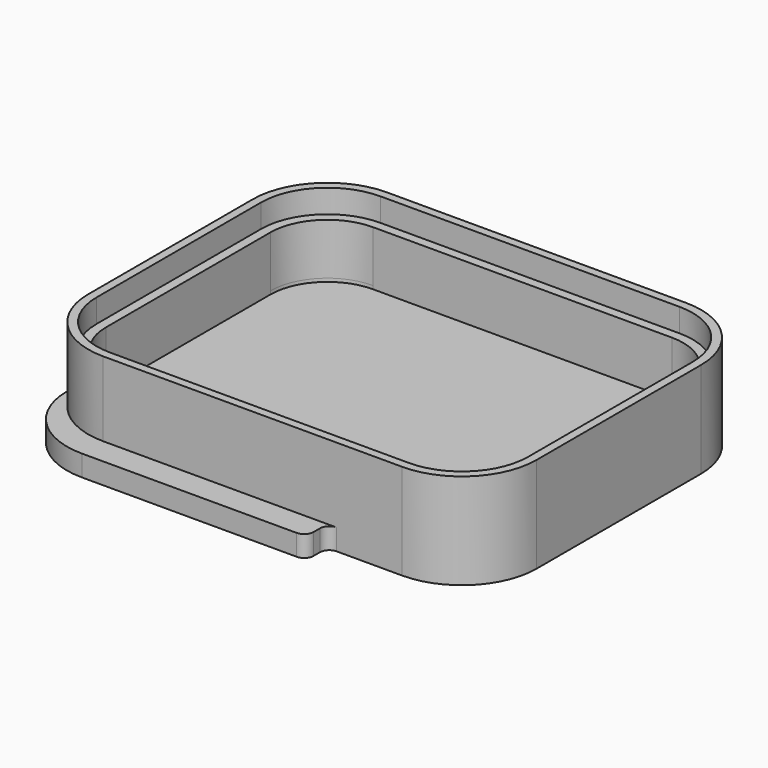
from build123d import *

# Parameters (mm, degrees)
F1_DEPTH     = 10.25
F3_DEPTH     = 2.25
F4_R         = 1
F5_T         = 1.9
F5_T3_DEPTH  = 4.8
F5_T5_DEPTH  = 27.8
F5_T8_ANGLE  = 90.000000001
F5_T10_ANGLE = 90.000000001
F7_DEPTH     = 2.5


# Not quite as in the source:
# - a shell that OpenCascade refuses in one call is made with other operations: the cavity is built on its own and cut out


with BuildPart() as f1:
    # F0 (on Top) → F1 (new body)
    with BuildSketch(Plane.XY):
        with BuildLine():
            Line((16, 19), (-16, 19))
            ThreePointArc((-16, 19), (-21.6568542495, 16.6568542495), (-24, 11))
            Line((-24, 11), (-24, -11))
            ThreePointArc((-24, -11), (-21.6568542495, -16.6568542495), (-16, -19))
            Line((-16, -19), (16, -19))
            ThreePointArc((16, -19), (21.6568542495, -16.6568542495), (24, -11))
            Line((24, -11), (24, 11))
            ThreePointArc((24, 11), (21.6568542495, 16.6568542495), (16, 19))
        make_face()
    extrude(amount=F1_DEPTH)

    # F2 (on Top) → F3 (join)
    with BuildSketch(Plane.XY):
        with BuildLine():
            Line((8, 21.85), (-16, 21.85))
            ThreePointArc((-16, 21.85), (-21.6568542495, 19.5068542495), (-24, 13.85))
            Line((-24, 13.85), (-24, -13.85))
            ThreePointArc((-24, -13.85), (-21.6568542495, -19.5068542495), (-16, -21.85))
            Line((-16, -21.85), (8, -21.85))
            Line((8, -21.85), (8, 21.85))
        make_face()
    extrude(amount=F3_DEPTH)

    # F4
    f4_edges = [f1.edges().sort_by_distance(p)[0] for p in [
        (8, 21.85, 1.125),
        (8, 19, 1.125),
        (8, -19, 1.125),
        (8, -21.85, 1.125),
    ]]
    fillet(f4_edges, radius=F4_R)

    # F5: shell of thickness 1.9, made by hand


with BuildPart() as f5_core1:
    # F5_t2: copy of F1
    add(f1.part)

    # the walls: a layer under each face that stays
    f5_faces = [f5_core1.faces().sort_by_distance(p)[0] for p in [
        (0, 19, 5.125),
        (0, 0, 0),
        (8.2928932188, 19.2928932188, 1.125),
        (21.6568542495, 16.6568542495, 5.125),
        (-18.5, 20.0416666667, 2.25),
        (-21.6568542495, 16.6568542495, 6.25),
        (8, 20.425, 1.125),
        (24, 0, 5.125),
        (21.6568542495, -16.6568542495, 5.125),
        (-4.5, 21.85, 1.125),
        (0, -19, 5.125),
        (-21.6568542495, 19.5068542495, 1.125),
        (8.2928932188, -19.2928932188, 1.125),
        (-24, 0, 5.125),
        (8, -20.425, 1.125),
        (-21.6568542495, -19.5068542495, 1.125),
        (-4.5, -21.85, 1.125),
        (-21.6568542495, -16.6568542495, 6.25),
        (-18.5, -20.0416666667, 2.25),
    ]]
    thicken(f5_faces, amount=-F5_T, mode=Mode.SUBTRACT)

    # F5_s4 → F5_t3 (cut)
    with BuildSketch(Plane.YZ.offset(6.1)):
        Polygon((19.019, 2.269), (17.1, 2.25), (17.1, 0.35), (19, 0.35), align=None)
        Polygon((-19.019, 2.269), (-17.1, 2.25), (-17.1, 0.35), (-19, 0.35), align=None)
    extrude(amount=F5_T3_DEPTH, mode=Mode.SUBTRACT)

    # F5_s6 → F5_t5 (cut)
    with BuildSketch(Plane.YZ.offset(-17.9)):
        Polygon((19.019, 2.269), (17.1, 2.25), (17.1, 0.35), (19, 0.35), align=None)
        Polygon((-19.019, 2.269), (-17.1, 2.25), (-17.1, 0.35), (-19, 0.35), align=None)
    extrude(amount=F5_T5_DEPTH, mode=Mode.SUBTRACT)

    # F5_s7 → F5_t8 (revolve, cut)
    with BuildSketch(Plane.XZ.offset(-11)):
        Polygon((-24.019, 2.269), (-24, 0.35), (-22.1, 0.35), (-22.1, 2.25), align=None)
    revolve(axis=Axis((-16, 11, 2.25), (0, 0, -1)), revolution_arc=F5_T8_ANGLE, mode=Mode.SUBTRACT)

    # F5_s9 → F5_t10 (revolve, cut)
    with BuildSketch(Plane.YZ.offset(-16)):
        Polygon((-19.019, 2.269), (-17.1, 2.25), (-17.1, 0.35), (-19, 0.35), align=None)
    revolve(axis=Axis((-16, -11, 2.25), (0, 0, -1)), revolution_arc=F5_T10_ANGLE, mode=Mode.SUBTRACT)


with BuildPart() as f1_1:
    add(f1.part)

    # what is left inside the walls is the cavity
    f5_cavity = [f5_core1.part.solids().sort_by_distance(p)[0] for p in [
        (0, -5.7, 10.231),
    ]]
    add(f5_cavity, mode=Mode.SUBTRACT)

    # F6 (on face) → F7 (cut)
    with BuildSketch(Plane.XY.offset(10.25)):
        with BuildLine():
            Line((23.1, -11), (23.1, 11))
            ThreePointArc((23.1, 11), (21.0204581464, 16.0204581464), (16, 18.1))
            Line((16, 18.1), (-16, 18.1))
            ThreePointArc((-16, 18.1), (-21.0204581464, 16.0204581464), (-23.1, 11))
            Line((-23.1, 11), (-23.1, -11))
            ThreePointArc((-23.1, -11), (-21.0204581464, -16.0204581464), (-16, -18.1))
            Line((-16, -18.1), (16, -18.1))
            ThreePointArc((16, -18.1), (21.0204581464, -16.0204581464), (23.1, -11))
        make_face()
        with BuildLine():
            Line((-22.1, -11), (-22.1, 11))
            ThreePointArc((-22.1, 11), (-20.3133513652, 15.3133513652), (-16, 17.1))
            Line((-16, 17.1), (16, 17.1))
            ThreePointArc((16, 17.1), (20.3133513652, 15.3133513652), (22.1, 11))
            Line((22.1, 11), (22.1, -11))
            ThreePointArc((22.1, -11), (20.3133513652, -15.3133513652), (16, -17.1))
            Line((16, -17.1), (-16, -17.1))
            ThreePointArc((-16, -17.1), (-20.3133513652, -15.3133513652), (-22.1, -11))
        make_face(mode=Mode.SUBTRACT)
    extrude(amount=-F7_DEPTH, mode=Mode.SUBTRACT)


solid = f1_1.part
